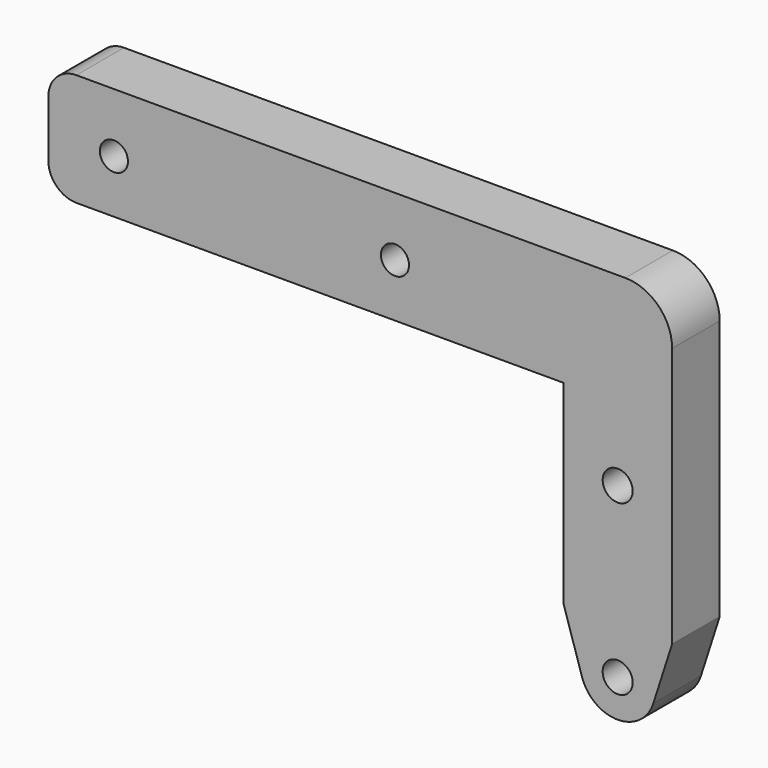
from build123d import *

# Parameters (mm, degrees)
F1_DEPTH = 6.35
F2_R     = 1.5
F2_R_2   = 1.6
F3_DEPTH = 6.351
F5_DEPTH = 3
F6_R     = 2.99999


# Not quite as in the source:
# - a fillet or chamfer is up to 0.001 mm smaller than in the source, because OpenCascade refuses the exact size


with BuildPart() as f1:
    # F0 (on Front) → F1 (new body)
    with BuildSketch(Plane.XZ):
        with BuildLine():
            Line((33, 6.3125771578), (-19, 6.3125771578))
            ThreePointArc((-19, 6.3125771578), (-21.1213203436, 5.4338975014), (-22, 3.3125771578))
            Line((-22, 3.3125771578), (-22, -2.6874228422))
            ThreePointArc((-22, -2.6874228422), (-21.1213203436, -4.8087431858), (-19, -5.6874228422))
            Line((-19, -5.6874228422), (33, -5.6874228422))
            Line((33, -5.6874228422), (33, -18.461904466))
            Line((33, -18.461904466), (33, -26.461904466))
            Line((33, -26.461904466), (34.9491434073, -32.6615871174))
            ThreePointArc((34.9491434073, -32.6615871174), (38.7515149865, -35.4618817353), (42.5726810332, -32.6872881404))
            Line((42.5726810332, -32.6872881404), (44.5761270821, -26.461904466))
            Line((44.5761270821, -26.461904466), (44.5761270821, -18.461904466))
            Line((44.5761270821, -18.461904466), (44.5761270821, 1.3125771578))
            ThreePointArc((44.5761270821, 1.3125771578), (43.111660988, 4.8481110637), (39.5761270821, 6.3125771578))
            Line((39.5761270821, 6.3125771578), (33, 6.3125771578))
        make_face()
    extrude(amount=F1_DEPTH)

    # F2 (on face) → F3 (cut, through all)
    with BuildSketch(Plane.XZ):
        with Locations((-15, 0)):
            Circle(F2_R)
        with Locations((15, 0)):
            Circle(F2_R)
        with Locations((38.765, -13.461904466)):
            Circle(F2_R_2)
        with Locations((38.765, -31.461904466)):
            Circle(F2_R_2)
    extrude(amount=F3_DEPTH, mode=Mode.SUBTRACT)

    # F4 (on face) → F5 (join)
    with BuildSketch(Plane.XZ):
        Polygon((41.4565890705, -5.352164329), (32.2204606053, 2.3090321163), (30.305161494, 0), (39.5412899592, -7.6611964453), align=None)
    extrude(amount=-F5_DEPTH)

    # F6 (radius 3 in the source; OpenCascade refuses exactly that, so slightly less here)
    f6_edges = [f1.edges().sort_by_distance(p)[0] for p in [
        (31.262811, 3, 1.154516),
        (40.49894, 3, -6.50668),
    ]]
    fillet(f6_edges, radius=F6_R)


solid = f1.part
